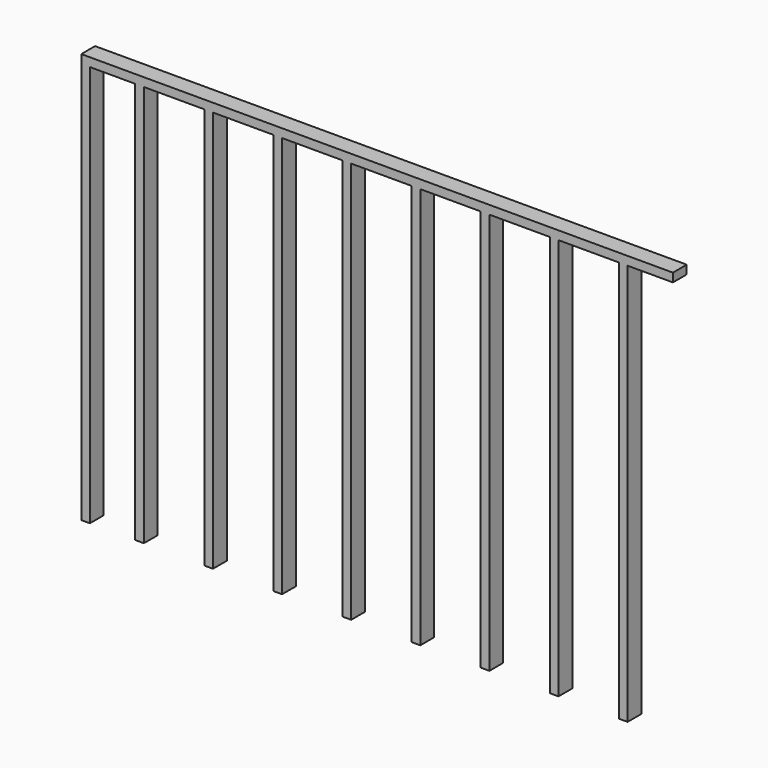
from build123d import *

# Parameters (mm, degrees)
F0_W     = 50.8
F0_H     = 2362.2
F1_DEPTH = 101.6
F2_W     = 101.6
F2_H     = 50.8
F3_DEPTH = 3479.8
F4_W     = 50.8
F4_H     = 101.6
F5_DEPTH = 2362.2


# Not quite as in the source:
# - a feature names something its author has since deleted; it is built from what else it names


with BuildPart() as f1:
    # F0 (on Front) → F1 (new body)
    with BuildSketch(Plane.XZ):
        with Locations((-51.6230743378, 769.2967753548)):
            Rectangle(F0_W, F0_H)
    extrude(amount=F1_DEPTH)

    # F2 (on face) → F3 (join)
    with BuildSketch(Plane(origin=(-77.0230743378, 0, 0), x_dir=(0, -1, 0), z_dir=(-1, 0, 0))):
        with Locations((50.8, 1975.7967753548)):
            Rectangle(F2_W, F2_H)
    extrude(amount=-F3_DEPTH)

    # F4 (on face) → F5 (join)
    with BuildSketch(Plane(origin=(0, 0, 1950.3967753548), x_dir=(1, 0, 0), z_dir=(0, 0, -1))):
        with Locations((265.8769256622, 50.8)):
            Rectangle(F4_W, F4_H)
        with Locations((672.2769256622, 50.8)):
            Rectangle(F4_W, F4_H)
        with Locations((1078.6769256622, 50.8)):
            Rectangle(F4_W, F4_H)
        with Locations((1485.0769256622, 50.8)):
            Rectangle(F4_W, F4_H)
        with Locations((1891.4769256622, 50.8)):
            Rectangle(F4_W, F4_H)
        with Locations((2297.8769256622, 50.8)):
            Rectangle(F4_W, F4_H)
        with Locations((2704.2769256622, 50.8)):
            Rectangle(F4_W, F4_H)
        with Locations((3110.6769256622, 50.8)):
            Rectangle(F4_W, F4_H)
    extrude(amount=F5_DEPTH)


solid = f1.part
